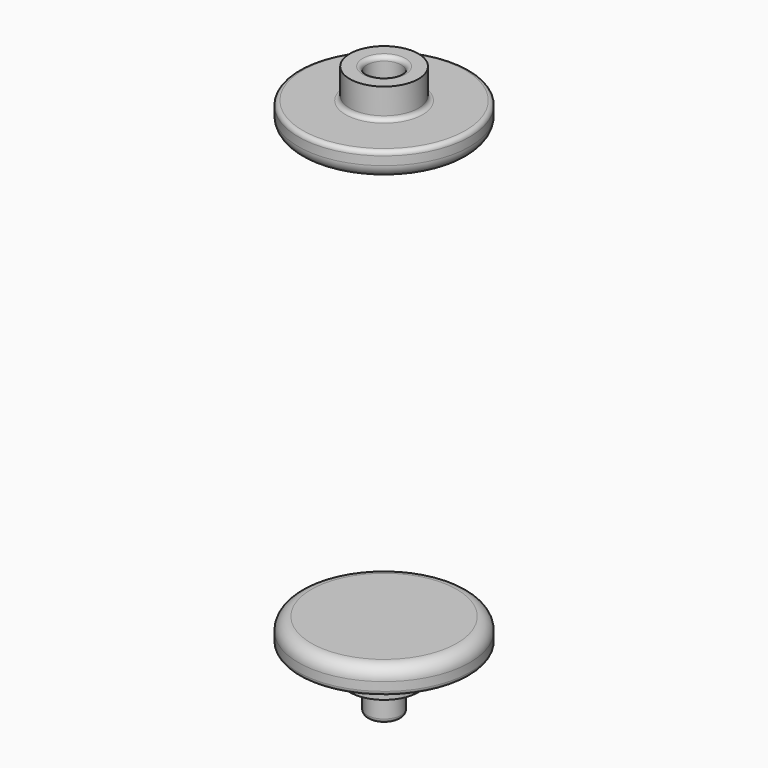
from build123d import *

# Parameters (mm, degrees)
F0_R     = 10
F0_R_2   = 4
F1_DEPTH = 3
F2_DEPTH = 3.5
F5_R     = 2
F6_DEPTH = 3.5
F8_D     = 4
F8_DEPTH = 3.5
F8_TIP   = 1.2017212381
F9_R     = 0.5
F9_2_R   = 0.5
F10_R    = 1.5
F10_2_R  = 1.5


with BuildPart() as f1:
    # F0 (on Top) → F1 (new body)
    with BuildSketch(Plane.XY):
        Circle(F0_R)
        Circle(F0_R_2, mode=Mode.SUBTRACT)
        Circle(F0_R_2)
    extrude(amount=F1_DEPTH)

    # F0 (on Top) → F2 (join)
    with BuildSketch(Plane.XY):
        Circle(F0_R_2)
    extrude(amount=-F2_DEPTH)


with BuildPart() as f4_1:
    # F4: instance of F1
    add(f1.part.mirror(Plane.XY.offset(28)))

    # F8
    with Locations(Plane.XY.offset(59.5)):
        with Locations((0, 0)):
            Hole(F8_D / 2, depth=F8_DEPTH)
            with Locations((0, 0, -(F8_DEPTH + F8_TIP / 2))):  # 118° drill point
                Cone(0, F8_D / 2, F8_TIP, mode=Mode.SUBTRACT)

    # F9#2
    f9_2_edges = [f4_1.edges().sort_by_distance(p)[0] for p in [
        (-10, 0, 56),
        (-4, 0, 56),
        (-2, 0, 59.5),
    ]]
    fillet(f9_2_edges, radius=F9_2_R)

    # F10#2
    f10_2_edges = [f4_1.edges().sort_by_distance(p)[0] for p in [
        (-10, 0, 53),
    ]]
    fillet(f10_2_edges, radius=F10_2_R)


with BuildPart() as f1_1:
    add(f1.part)

    # F5 (on face) → F6 (join)
    with BuildSketch(Plane(origin=(0, 0, -3.5), x_dir=(1, 0, 0), z_dir=(0, 0, -1))):
        Circle(F5_R)
    extrude(amount=F6_DEPTH)

    # F9
    f9_edges = [f1_1.edges().sort_by_distance(p)[0] for p in [
        (-2, 0, -7),
        (-2, 0, -3.5),
        (-4, 0, 0),
        (-10, 0, 0),
    ]]
    fillet(f9_edges, radius=F9_R)

    # F10
    f10_edges = [f1_1.edges().sort_by_distance(p)[0] for p in [
        (-10, 0, 3),
    ]]
    fillet(f10_edges, radius=F10_R)


solid = Compound([f4_1.part, f1_1.part])
